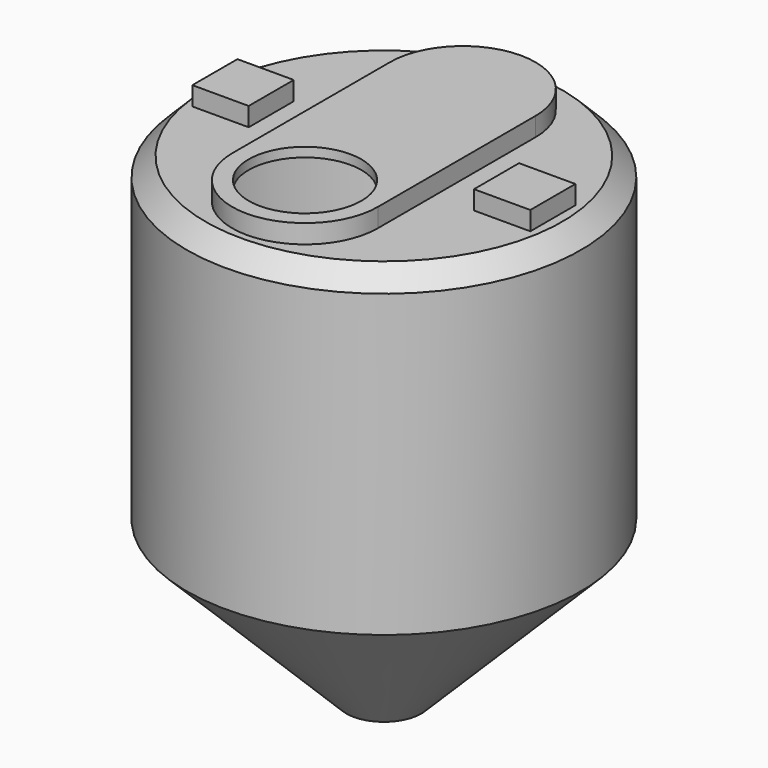
from build123d import *

# Parameters (mm, degrees)
F2_W         = 152.4
F2_H         = 152.4
F3_DEPTH     = 50.8
F5_DEPTH     = 50.8
F6_R         = 152.4
F7_DEPTH     = 25.4
F8_T         = 6.35
F8_T3_DEPTH  = 165.1
F8_T5_DEPTH  = 165.1
F8_T7_DEPTH  = 546.1
F8_T9_DEPTH  = 165.1
F8_T12_ANGLE = 180.000000001
F8_T14_ANGLE = 180.000000001
F9_W         = 101.6
F9_H         = 101.6
F9_R         = 25.4
F10_DEPTH    = 38.1
F11_R        = 19.05


# Not quite as in the source:
# - a pattern or mirror of a feature is missing from the dataset's text; its kind, count and spacing are read off the source's solid
# - a shell that OpenCascade refuses in one call is made with other operations: the cavity is built on its own and cut out


with BuildPart() as f1:
    # F0 (on Front) → F1 (revolve)
    with BuildSketch(Plane.XZ):
        Polygon((-101.6, 0), (0, 0), (0, 1295.4), (-482.6, 1295.4), (-533.4, 1244.6), (-533.4, 431.8), align=None)
    revolve(axis=Axis((0, 0, 647.7), (0, 0, -1)))

    # F2 (on face) → F3 (join)
    with BuildSketch(Plane.XY.offset(1295.4)):
        with Locations((381, 0)):
            Rectangle(F2_W, F2_H)
    f3 = extrude(amount=F3_DEPTH)

    # F3_copies: F3 across plane
    add(f3.mirror(Plane(origin=(0, 0, 0), x_dir=(0, 0, -1), z_dir=(-1, 0, 0))))

    # F4 (on face) → F5 (join)
    with BuildSketch(Plane.XY.offset(1295.4)):
        with BuildLine():
            ThreePointArc((0, 463.55), (-139.1939698766, 405.8939698766), (-196.85, 266.7))
            Line((-196.85, 266.7), (-196.85, -266.7))
            ThreePointArc((-196.85, -266.7), (-139.1939698766, -405.8939698766), (0, -463.55))
            ThreePointArc((0, -463.55), (139.1939698766, -405.8939698766), (196.85, -266.7))
            Line((196.85, -266.7), (196.85, 266.7))
            ThreePointArc((196.85, 266.7), (139.1939698766, 405.8939698766), (0, 463.55))
        make_face()
    extrude(amount=F5_DEPTH)

    # F6 (on face) → F7 (cut)
    with BuildSketch(Plane.XY.offset(1346.2)):
        with Locations((0, -266.7)):
            Circle(F6_R)
    extrude(amount=-F7_DEPTH, mode=Mode.SUBTRACT)

    # F8: shell of thickness 6.35, made by hand


with BuildPart() as f8_core1:
    # F8_t2: copy of F1
    add(f1.part)

    # the walls: a layer under each face that stays
    f8_faces = [f8_core1.faces().sort_by_distance(p)[0] for p in [
        (0, 0, 0),
        (317.5, 0, 215.9),
        (533.4, 0, 838.2),
        (508, 0, 1270),
        (-321.7333333333, -321.7333333333, 1295.4),
        (-457.2, 0, 1320.8),
        (-381, -76.2, 1320.8),
        (-381, 76.2, 1320.8),
        (-304.8, 0, 1320.8),
        (0, 463.55, 1320.8),
        (-196.85, 0, 1320.8),
        (0, -463.55, 1320.8),
        (196.85, 0, 1320.8),
        (381, 76.2, 1320.8),
        (457.2, 0, 1320.8),
        (304.8, 0, 1320.8),
        (381, -76.2, 1320.8),
        (-381, 0, 1346.2),
        (0, 0, 1346.2),
        (381, 0, 1346.2),
        (-152.4, -266.7, 1333.5),
    ]]
    thicken(f8_faces, amount=-F8_T, mode=Mode.SUBTRACT)

    # F8_s4 → F8_t3 (cut)
    with BuildSketch(Plane.XZ.offset(-82.55)):
        Polygon((-457.2635, 1295.4635), (-457.2, 1289.05), (-450.85, 1289.05), (-450.85, 1295.4), align=None)
        Polygon((-304.7365, 1295.4635), (-304.8, 1289.05), (-311.15, 1289.05), (-311.15, 1295.4), align=None)
        Polygon((457.2635, 1295.4635), (457.2, 1289.05), (450.85, 1289.05), (450.85, 1295.4), align=None)
        Polygon((304.7365, 1295.4635), (304.8, 1289.05), (311.15, 1289.05), (311.15, 1295.4), align=None)
    extrude(amount=F8_T3_DEPTH, mode=Mode.SUBTRACT)

    # F8_s6 → F8_t5 (cut)
    with BuildSketch(Plane.YZ.offset(-463.55)):
        Polygon((-76.2635, 1295.4635), (-76.2, 1289.05), (-69.85, 1289.05), (-69.85, 1295.4), align=None)
        Polygon((76.2635, 1295.4635), (76.2, 1289.05), (69.85, 1289.05), (69.85, 1295.4), align=None)
    extrude(amount=F8_T5_DEPTH, mode=Mode.SUBTRACT)

    # F8_s8 → F8_t7 (cut)
    with BuildSketch(Plane.XZ.offset(-273.05)):
        Polygon((-196.9135, 1295.4635), (-196.85, 1289.05), (-190.5, 1289.05), (-190.5, 1295.4), align=None)
        Polygon((196.9135, 1295.4635), (196.85, 1289.05), (190.5, 1289.05), (190.5, 1295.4), align=None)
    extrude(amount=F8_T7_DEPTH, mode=Mode.SUBTRACT)

    # F8_s10 → F8_t9 (cut)
    with BuildSketch(Plane.YZ.offset(298.45)):
        Polygon((76.2635, 1295.4635), (76.2, 1289.05), (69.85, 1289.05), (69.85, 1295.4), align=None)
        Polygon((-76.2635, 1295.4635), (-76.2, 1289.05), (-69.85, 1289.05), (-69.85, 1295.4), align=None)
    extrude(amount=F8_T9_DEPTH, mode=Mode.SUBTRACT)

    # F8_s11 → F8_t12 (revolve, cut)
    with BuildSketch(Plane.XZ.offset(-266.7)):
        Polygon((196.9135, 1295.4635), (196.85, 1289.05), (190.5, 1289.05), (190.5, 1295.4), align=None)
    revolve(axis=Axis((0, 266.7, 1295.4), (0, 0, 1)), revolution_arc=F8_T12_ANGLE, mode=Mode.SUBTRACT)

    # F8_s13 → F8_t14 (revolve, cut)
    with BuildSketch(Plane.XZ.offset(266.7)):
        Polygon((-196.9135, 1295.4635), (-196.85, 1289.05), (-190.5, 1289.05), (-190.5, 1295.4), align=None)
    revolve(axis=Axis((0, -266.7, 1295.4), (0, 0, 1)), revolution_arc=F8_T14_ANGLE, mode=Mode.SUBTRACT)


with BuildPart() as f1_1:
    add(f1.part)

    # what is left inside the walls is the cavity
    f8_cavity = [f8_core1.part.solids().sort_by_distance(p)[0] for p in [
        (526.9865, 0, 972.789915),
    ]]
    add(f8_cavity, mode=Mode.SUBTRACT)

    # F9 (on face) → F10 (join)
    with BuildSketch(Plane.XY.offset(6.35)):
        Rectangle(F9_W, F9_H)
        Circle(F9_R, mode=Mode.SUBTRACT)
    extrude(amount=F10_DEPTH)

    # F11
    f11_edges = [f1_1.edges().sort_by_distance(p)[0] for p in [
        (-50.8, -50.8, 25.4),
        (50.8, -50.8, 25.4),
        (50.8, 50.8, 25.4),
        (-50.8, 50.8, 25.4),
    ]]
    fillet(f11_edges, radius=F11_R)


solid = f1_1.part
